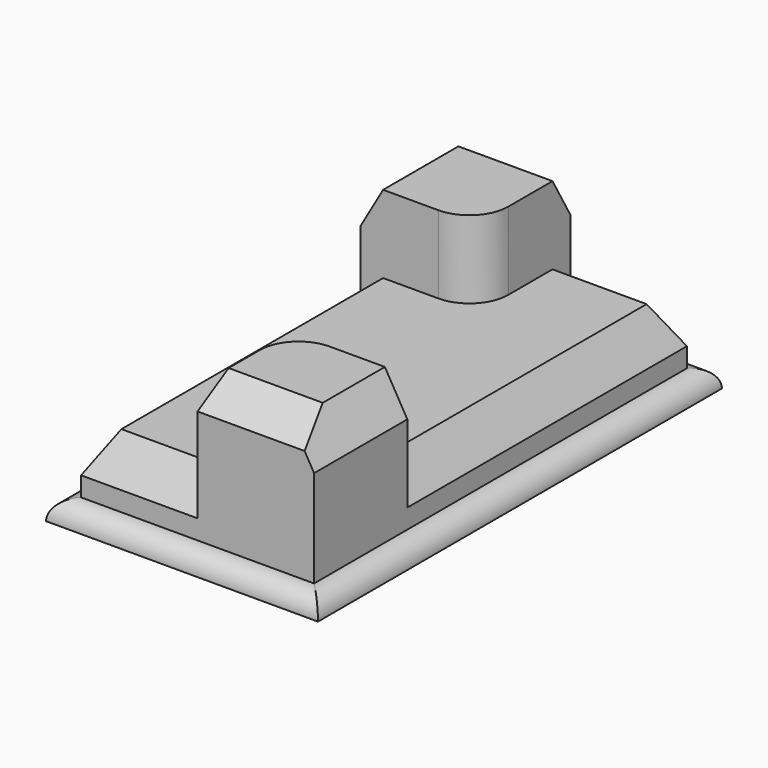
from build123d import *

# Parameters (mm, degrees)
F1_DEPTH    = 25.4
F2_DEPTH    = 50.8
F0_W        = 88.9
F0_H        = 165.1
F3_DEPTH    = 6.35
F4_R        = 6.34999
F5_SIZE2    = 7.3323484187
F5_SIZE     = 12.7
F6_C1_SIZE2 = 7.3323484187
F6_C1_SIZE  = 12.7
F6_C2_SIZE2 = 12.7
F6_C2_SIZE  = 7.3323484187
F6_C3_SIZE2 = 7.3323484187
F6_C3_SIZE  = 12.7
F6_C4_SIZE2 = 7.3323484187
F6_C4_SIZE  = 12.7


# Not quite as in the source:
# - a fillet or chamfer is up to 0.001 mm smaller than in the source, because OpenCascade refuses the exact size


with BuildPart() as f1:
    # F0 (on Top) → F1 (new body)
    with BuildSketch(Plane.XY):
        with BuildLine():
            Line((30.3925445665, 58.8535625324), (-7.7074554335, 58.8535625324))
            Line((-7.7074554335, 58.8535625324), (-7.7074554335, 33.4535625324))
            ThreePointArc((-7.7074554335, 33.4535625324), (-11.4271993125, 24.4733064113), (-20.4074554335, 20.7535625324))
            Line((-20.4074554335, 20.7535625324), (-45.8074554335, 20.7535625324))
            Line((-45.8074554335, 20.7535625324), (-45.8074554335, -93.5464374676))
            Line((-45.8074554335, -93.5464374676), (-7.7074554335, -93.5464374676))
            Line((-7.7074554335, -93.5464374676), (-7.7074554335, -68.1464374676))
            ThreePointArc((-7.7074554335, -68.1464374676), (-3.9877115546, -59.1661813466), (4.9925445665, -55.4464374676))
            Line((4.9925445665, -55.4464374676), (30.3925445665, -55.4464374676))
            Line((30.3925445665, -55.4464374676), (30.3925445665, 58.8535625324))
        make_face()
    extrude(amount=F1_DEPTH)

    # F0 (on Top) → F2 (join)
    with BuildSketch(Plane.XY):
        with BuildLine():
            Line((-7.7074554335, 58.8535625324), (-45.8074554335, 58.8535625324))
            Line((-45.8074554335, 58.8535625324), (-45.8074554335, 20.7535625324))
            Line((-45.8074554335, 20.7535625324), (-20.4074554335, 20.7535625324))
            ThreePointArc((-20.4074554335, 20.7535625324), (-11.4271993125, 24.4733064113), (-7.7074554335, 33.4535625324))
            Line((-7.7074554335, 33.4535625324), (-7.7074554335, 58.8535625324))
        make_face()
        with BuildLine():
            Line((30.3925445665, -93.5464374676), (30.3925445665, -55.4464374676))
            Line((30.3925445665, -55.4464374676), (4.9925445665, -55.4464374676))
            ThreePointArc((4.9925445665, -55.4464374676), (-3.9877115546, -59.1661813466), (-7.7074554335, -68.1464374676))
            Line((-7.7074554335, -68.1464374676), (-7.7074554335, -93.5464374676))
            Line((-7.7074554335, -93.5464374676), (30.3925445665, -93.5464374676))
        make_face()
    extrude(amount=F2_DEPTH)

    # F0 (on Top) → F3 (join)
    with BuildSketch(Plane.XY):
        with Locations((-7.7074554335, -17.3464374676)):
            Rectangle(F0_W, F0_H)
        Polygon((-45.8074554335, 20.7535625324), (-45.8074554335, 58.8535625324), (-7.7074554335, 58.8535625324), (30.3925445665, 58.8535625324), (30.3925445665, -55.4464374676), (30.3925445665, -93.5464374676), (-7.7074554335, -93.5464374676), (-45.8074554335, -93.5464374676), align=None, mode=Mode.SUBTRACT)
    extrude(amount=F3_DEPTH)

    # F4 (radius 6.35 in the source; OpenCascade refuses exactly that, so slightly less here)
    f4_edges = [f1.edges().sort_by_distance(p)[0] for p in [
        (-7.707455, -99.896437, 6.35),
        (-52.157455, -17.346437, 6.35),
        (36.742545, -17.346437, 6.35),
        (-7.707455, 65.203563, 6.35),
    ]]
    fillet(f4_edges, radius=F4_R)

    # F5
    f5_edges = [f1.edges().sort_by_distance(p)[0] for p in [
        (30.392545, 1.703563, 25.4),
        (11.342545, 58.853563, 25.4),
        (-45.807455, -36.396437, 25.4),
        (-26.757455, -93.546437, 25.4),
    ]]
    chamfer(f5_edges, length=F5_SIZE, length2=F5_SIZE2)

    # F6: chamfer of 12.7 x 7.3323484187 on 4 edges, made by hand

    # F6_c1
    f6_c1_edges = [f1.edges().sort_by_distance(p)[0] for p in [
        (-45.8074554335, 39.8035625324, 50.8),
    ]]
    f6_c1_side = f1.faces().sort_by_distance((-45.8074554335, 39.8035625324, 50.6533530316))[0]
    chamfer(f6_c1_edges, length=F6_C1_SIZE, length2=F6_C1_SIZE2, reference=f6_c1_side)

    # F6_c2
    f6_c2_edges = [f1.edges().sort_by_distance(p)[0] for p in [
        (11.3425445665, -93.5464374676, 50.8),
    ]]
    f6_c2_side = f1.faces().sort_by_distance((11.3425445665, -93.5464374676, 50.6533530316))[0]
    chamfer(f6_c2_edges, length=F6_C2_SIZE, length2=F6_C2_SIZE2, reference=f6_c2_side)

    # F6_c3
    f6_c3_edges = [f1.edges().sort_by_distance(p)[0] for p in [
        (-23.0912812242, 58.8535625324, 50.8),
    ]]
    f6_c3_side = f1.faces().sort_by_distance((-23.0912812242, 58.8535625324, 50.6533530316))[0]
    chamfer(f6_c3_edges, length=F6_C3_SIZE, length2=F6_C3_SIZE2, reference=f6_c3_side)

    # F6_c4
    f6_c4_edges = [f1.edges().sort_by_distance(p)[0] for p in [
        (30.3925445665, -68.1464374676, 50.8),
    ]]
    f6_c4_side = f1.faces().sort_by_distance((30.3925445665, -68.1464374676, 50.6533530316))[0]
    chamfer(f6_c4_edges, length=F6_C4_SIZE, length2=F6_C4_SIZE2, reference=f6_c4_side)


solid = f1.part
